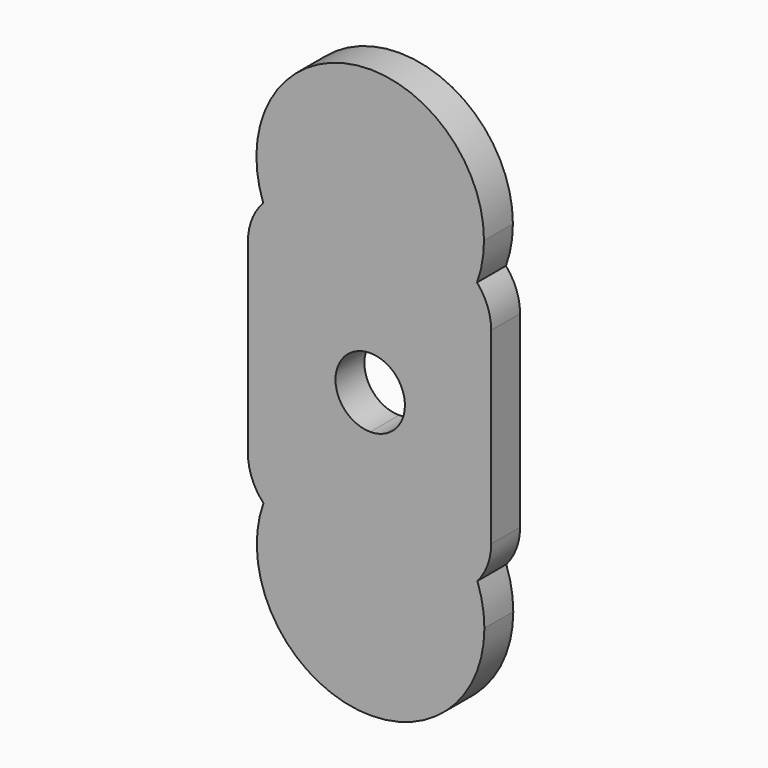
from build123d import *

# Parameters (mm, degrees)
F1_DEPTH = 3.175


# Not quite as in the source:
# - a feature names something its author has since deleted; it is built from what else it names


with BuildPart() as f1:
    # F0 (on Front) → F1 (new body)
    with BuildSketch(Plane.XZ):
        with BuildLine():
            ThreePointArc((0, 3.05), (2.1566756826, 2.1566756826), (3.05, 0))
            ThreePointArc((3.05, 0), (2.1566756826, -2.1566756826), (0, -3.05))
            Line((0, -3.05), (0, -4.9800602682))
            ThreePointArc((0, -4.9800602682), (5.7417944409, -6.7685559702), (9.4194688927, -11.5268782485))
            ThreePointArc((9.4194688927, -11.5268782485), (10.31824899, -10.0042357535), (10.6308735731, -8.2639737901))
            Line((10.6308735731, -8.2639737901), (10.6308735731, 8.2639737901))
            ThreePointArc((10.6308735731, 8.2639737901), (10.3103808484, 10.0252834336), (9.389988909, 11.5607983065))
            ThreePointArc((9.389988909, 11.5607983065), (5.7274768906, 6.8026828494), (0, 5))
            Line((0, 5), (0, 3.05))
        make_face()
        with BuildLine():
            ThreePointArc((0, -3.05), (-3.05, 0), (0, 3.05))
            Line((0, 3.05), (0, 5))
            ThreePointArc((0, 5), (-5.7423447428, 6.8130911295), (-9.4024106226, 11.5949046291))
            ThreePointArc((-9.4024106226, 11.5949046291), (-10.3983579477, 10.0170839844), (-10.7465008538, 8.183992176))
            Line((-10.7465008538, 8.183992176), (-10.7465008538, -8.183992176))
            ThreePointArc((-10.7465008538, -8.183992176), (-10.3930329558, -10.0305401514), (-9.3826050837, -11.6160099542))
            ThreePointArc((-9.3826050837, -11.6160099542), (-5.739751248, -6.8156278258), (0, -4.9800602682))
            Line((0, -4.9800602682), (0, -3.05))
        make_face()
        with BuildLine():
            ThreePointArc((-9.4024106226, 11.5949046291), (-5.7423447428, 6.8130911295), (0, 5))
            Line((0, 5), (0, 15))
            ThreePointArc((0, 15), (-4.5199654888, 14.3027938523), (-8.6197512808, 12.275988264))
            ThreePointArc((-8.6197512808, 12.275988264), (-9.0287945556, 11.9558018286), (-9.4024106226, 11.5949046291))
        make_face()
        with BuildLine():
            Line((0, 15), (0, 5))
            ThreePointArc((0, 5), (5.7274768906, 6.8026828494), (9.389988909, 11.5607983065))
            ThreePointArc((9.389988909, 11.5607983065), (8.9445660683, 12.0082283284), (8.4463103597, 12.3959606852))
            ThreePointArc((8.4463103597, 12.3959606852), (4.4193093195, 14.3342144933), (0, 15))
        make_face()
        with BuildLine():
            ThreePointArc((9.4194688927, -11.5268782485), (5.7417944409, -6.7685559702), (0, -4.9800602682))
            Line((0, -4.9800602682), (0, -15))
            ThreePointArc((0, -15), (4.4193093195, -14.3342144933), (8.4463103597, -12.3959606852))
            ThreePointArc((8.4463103597, -12.3959606852), (8.9613594363, -11.9932986506), (9.4194688927, -11.5268782485))
        make_face()
        with BuildLine():
            Line((0, -15), (0, -4.9800602682))
            ThreePointArc((0, -4.9800602682), (-5.739751248, -6.8156278258), (-9.3826050837, -11.6160099542))
            ThreePointArc((-9.3826050837, -11.6160099542), (-9.0178640795, -11.9652859553), (-8.6197512808, -12.275988264))
            ThreePointArc((-8.6197512808, -12.275988264), (-4.5199654888, -14.3027938523), (0, -15))
        make_face()
        with BuildLine():
            ThreePointArc((-8.6197512808, 12.275988264), (-4.5199654888, 14.3027938523), (0, 15))
            ThreePointArc((0, 15), (4.4193093195, 14.3342144933), (8.4463103597, 12.3959606852))
            ThreePointArc((8.4463103597, 12.3959606852), (8.9445660683, 12.0082283284), (9.389988909, 11.5607983065))
            ThreePointArc((9.389988909, 11.5607983065), (9.8463162932, 13.2535592037), (10, 15))
            ThreePointArc((10, 15), (-1.7285678717, 24.8494696869), (-9.4024106226, 11.5949046291))
            ThreePointArc((-9.4024106226, 11.5949046291), (-9.0287945556, 11.9558018286), (-8.6197512808, 12.275988264))
        make_face()
        with BuildLine():
            ThreePointArc((8.4463103597, -12.3959606852), (4.4193093195, -14.3342144933), (0, -15))
            ThreePointArc((0, -15), (-4.5199654888, -14.3027938523), (-8.6197512808, -12.275988264))
            ThreePointArc((-8.6197512808, -12.275988264), (-9.0178640795, -11.9652859553), (-9.3826050837, -11.6160099542))
            ThreePointArc((-9.3826050837, -11.6160099542), (-1.6724608086, -24.8332220833), (10.0345902517, -14.9800004438))
            ThreePointArc((10.0345902517, -14.9800004438), (9.8796089518, -13.2262596432), (9.4194688927, -11.5268782485))
            ThreePointArc((9.4194688927, -11.5268782485), (8.9613594363, -11.9932986506), (8.4463103597, -12.3959606852))
        make_face()
    extrude(amount=F1_DEPTH)


solid = f1.part
